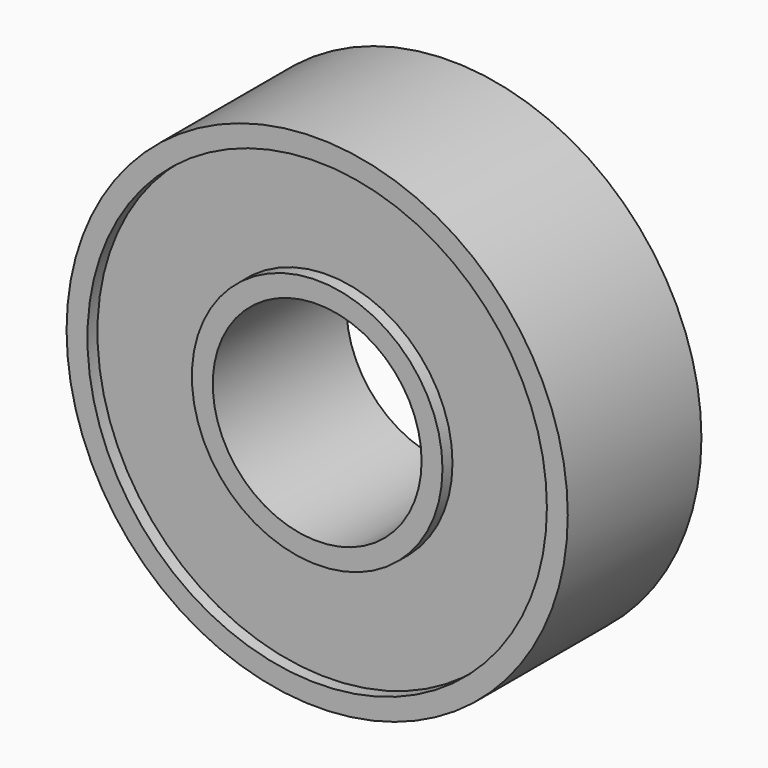
from build123d import *

# Parameters (mm, degrees)
F0_R     = 6
F0_R_2   = 2.5
F1_DEPTH = 2
F2_R     = 5.5
F2_R_2   = 3
F3_DEPTH = 0.3


# Not quite as in the source:
# - a pattern or mirror of a feature is missing from the dataset's text; its kind, count and spacing are read off the source's solid


with BuildPart() as f1:
    # F0 (on Front) → F1 (new body, symmetric)
    with BuildSketch(Plane.XZ):
        Circle(F0_R)
        Circle(F0_R_2, mode=Mode.SUBTRACT)
    extrude(amount=F1_DEPTH, both=True)

    # F2 (on face) → F3 (cut)
    with BuildSketch(Plane.XZ.offset(2)):
        Circle(F2_R)
        Circle(F2_R_2, mode=Mode.SUBTRACT)
    f3 = extrude(amount=-F3_DEPTH, mode=Mode.SUBTRACT)

    # F3_copies: F3 across plane
    add(f3.mirror(Plane.ZX), mode=Mode.SUBTRACT)


solid = f1.part
